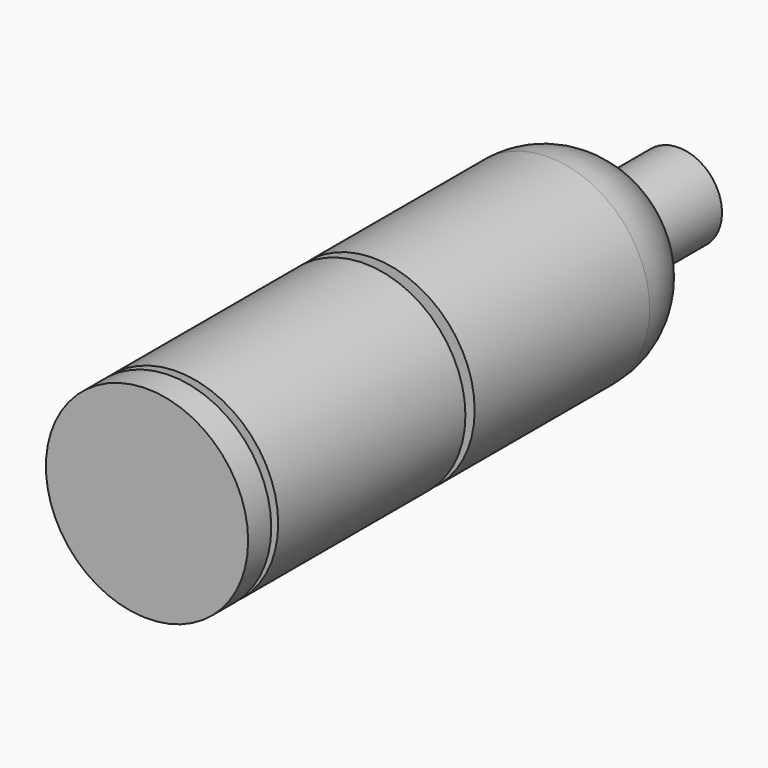
from build123d import *

# Parameters (mm, degrees)
F0_R     = 35
F1_DEPTH = 230
F3_R     = 40.5
F3_R_2   = 30.5
F4_DEPTH = 3
F6_R     = 40
F6_R_2   = 30.5
F7_DEPTH = 4
F8_R     = 40
F8_R_2   = 15
F9_DEPTH = 28


# Not quite as in the source:
# - a fillet or chamfer that OpenCascade refuses, or shapes differently, is made with other operations: its cross-section is extruded or revolved along the edge and cut away or added


with BuildPart() as f1:
    # F0 (on Front) → F1 (new body)
    with BuildSketch(Plane.XZ):
        Circle(F0_R)
    extrude(amount=-F1_DEPTH)

    # F3 (on offset) → F4 (cut)
    with BuildSketch(Plane.XZ.offset(-10)):
        Circle(F3_R)
        Circle(F3_R_2, mode=Mode.SUBTRACT)
    extrude(amount=-F4_DEPTH, mode=Mode.SUBTRACT)

    # F6 (on offset) → F7 (cut)
    with BuildSketch(Plane.XZ.offset(-94)):
        Circle(F6_R)
        Circle(F6_R_2, mode=Mode.SUBTRACT)
    extrude(amount=-F7_DEPTH, mode=Mode.SUBTRACT)

    # F8 (on face) → F9 (cut)
    with BuildSketch(Plane(origin=(0, 230, 0), x_dir=(-1, 0, 0), z_dir=(0, 1, 0))):
        Circle(F8_R)
        Circle(F8_R_2, mode=Mode.SUBTRACT)
    extrude(amount=-F9_DEPTH, mode=Mode.SUBTRACT)

    # F10: fillet of radius 30 on 1 edges, made by hand

    # F10_s1 → F10_t2 (revolve, cut)
    with BuildSketch(Plane.XY):
        with BuildLine():
            ThreePointArc((35, 173.7157287525), (29.4948974278, 191.0362368282), (15, 202))
            Line((15, 202), (35, 202))
            Line((35, 202), (35, 173.7157287525))
        make_face()
    revolve(axis=Axis((0, 202, 0), (0, -1, 0)), mode=Mode.SUBTRACT)


solid = f1.part
